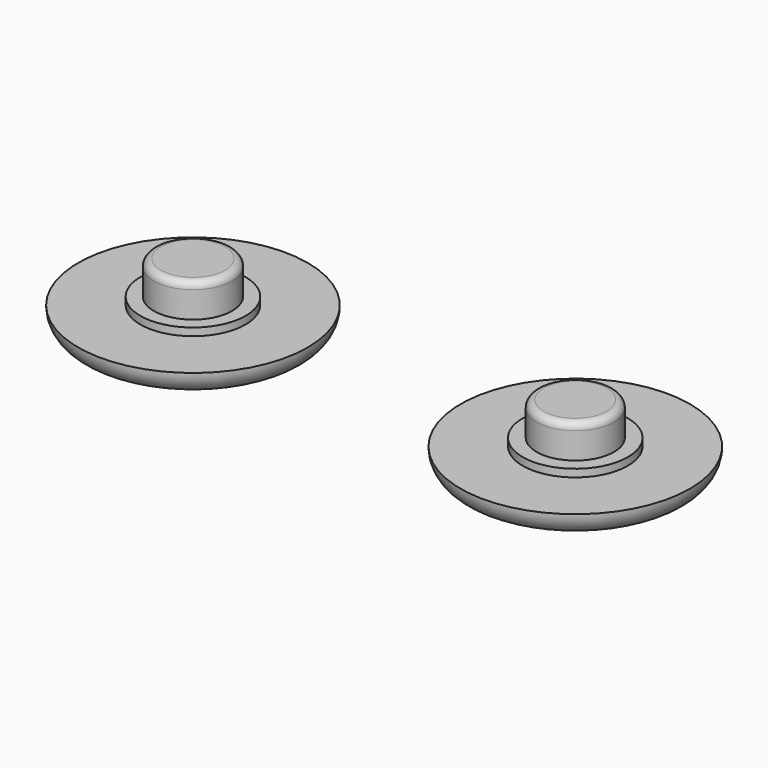
from build123d import *

# Parameters (mm, degrees)
F0_R     = 12
F1_DEPTH = 2.5
F2_R     = 5.5
F3_DEPTH = 0.8
F4_R     = 4.1
F5_DEPTH = 3.5
F4_R_2   = 4.05
F6_R     = 2.49999
F6_2_R   = 2.49999
F7_R     = 0.75
F7_2_R   = 0.75


# Not quite as in the source:
# - a fillet or chamfer is up to 0.001 mm smaller than in the source, because OpenCascade refuses the exact size


with BuildPart() as f1:
    # F0 (on Top) → F1 (new body)
    with BuildSketch(Plane.XY):
        Circle(F0_R)
    extrude(amount=F1_DEPTH)

    # F2 (on face) → F3 (join)
    with BuildSketch(Plane.XY.offset(2.5)):
        Circle(F2_R)
    extrude(amount=F3_DEPTH)

    # F4 (on face) → F5 (join)
    with BuildSketch(Plane.XY.offset(3.3)):
        Circle(F4_R)
    extrude(amount=F5_DEPTH)

    # F6 (radius 2.5 in the source; OpenCascade refuses exactly that, so slightly less here)
    f6_edges = [f1.edges().sort_by_distance(p)[0] for p in [
        (-12, 0, 0),
    ]]
    fillet(f6_edges, radius=F6_R)

    # F7
    f7_edges = [f1.edges().sort_by_distance(p)[0] for p in [
        (-4.1, 0, 6.8),
    ]]
    fillet(f7_edges, radius=F7_R)


with BuildPart() as f1b:
    # F0 (on Top) → F1, piece 2 (new body)
    with BuildSketch(Plane.XY):
        with Locations((40, 0)):
            Circle(F0_R)
    extrude(amount=F1_DEPTH)

    # F2 (on face) → F3, piece 2 (join)
    with BuildSketch(Plane.XY.offset(2.5)):
        with Locations((40, 0)):
            Circle(F2_R)
    extrude(amount=F3_DEPTH)

    # F4 (on face) → F5, piece 2 (join)
    with BuildSketch(Plane.XY.offset(3.3)):
        with Locations((40, 0)):
            Circle(F4_R_2)
    extrude(amount=F5_DEPTH)

    # F6#2 (radius 2.5 in the source; OpenCascade refuses exactly that, so slightly less here)
    f6_2_edges = [f1b.edges().sort_by_distance(p)[0] for p in [
        (28, 0, 0),
    ]]
    fillet(f6_2_edges, radius=F6_2_R)

    # F7#2
    f7_2_edges = [f1b.edges().sort_by_distance(p)[0] for p in [
        (35.95, 0, 6.8),
    ]]
    fillet(f7_2_edges, radius=F7_2_R)


solid = Compound([f1.part, f1b.part])
